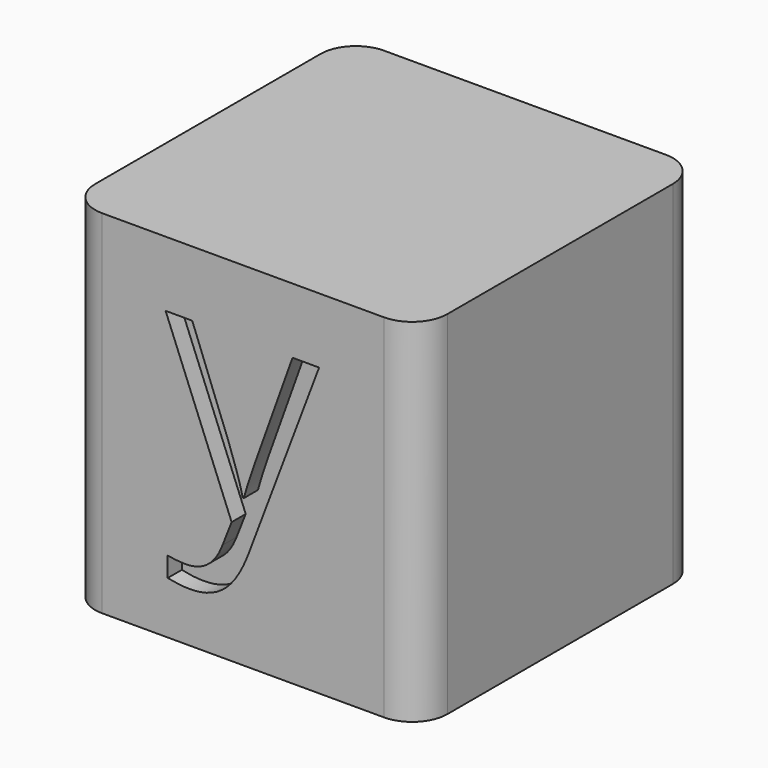
from build123d import *

# Parameters (mm, degrees)
F0_W         = 20
F0_H         = 20
F1_DEPTH     = 20
F2_R         = 2
F3_TEXT_SIZE = 25.098873367
F4_DEPTH     = 1
F5_TEXT_SIZE = 17.3611111111
F6_DEPTH     = 1


# Not quite as in the source:
# - Text() gives the source's letters only with a copy of the font that has no kerning and outlines rounded to 1/6400 em; it was checked with that copy


with BuildPart() as f1:
    # F0 (on Top) → F1 (new body)
    with BuildSketch(Plane.XY):
        Rectangle(F0_W, F0_H)
    extrude(amount=F1_DEPTH)

    # F2
    f2_edges = [f1.edges().sort_by_distance(p)[0] for p in [
        (-10, -10, 10),
        (-10, 10, 10),
        (10, -10, 10),
        (10, 10, 10),
    ]]
    fillet(f2_edges, radius=F2_R)

    # F3 (on face) → F4 (cut)
    with BuildSketch(Plane(origin=(-10, 0, 0), x_dir=(0, -1, 0), z_dir=(-1, 0, 0))):
        with Locations((-6.5651971963, 2.6371575659)):
            Text('x', F3_TEXT_SIZE, font='Open Sans', text_align=(TextAlign.LEFT, TextAlign.BOTTOM))
    extrude(amount=-F4_DEPTH, mode=Mode.SUBTRACT)

    # F5 (on face) → F6 (cut)
    with BuildSketch(Plane.XZ.offset(10)):
        with Locations((-4.4178559028, 7)):
            Text('y', F5_TEXT_SIZE, font='Open Sans', text_align=(TextAlign.LEFT, TextAlign.BOTTOM))
    extrude(amount=-F6_DEPTH, mode=Mode.SUBTRACT)


solid = f1.part
